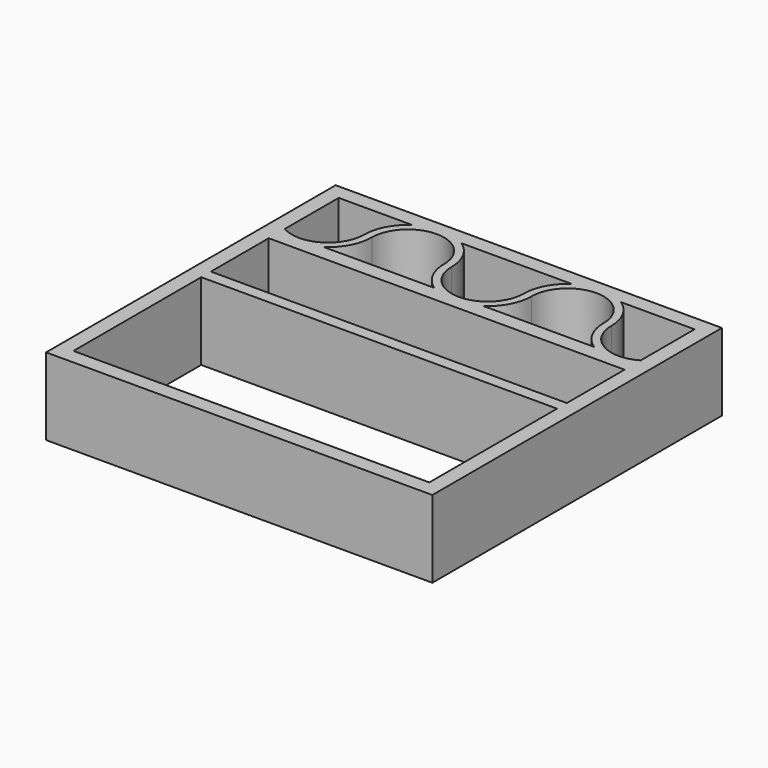
from build123d import *

# Parameters (mm, degrees)
F0_W     = 127
F0_H     = 119
F0_W_2   = 117
F0_H_2   = 23.75
F1_DEPTH = 25.4


# Not quite as in the source:
# - a feature of the source that left no trace in its solid (it failed there, or was rolled back) is left out


with BuildPart() as f1:
    # F0 (on Top) → F1 (new body)
    with BuildSketch(Plane.XY):
        Rectangle(F0_W, F0_H)
        Polygon((58.5, -54.5), (-58.5, -54.5), (-58.5, -30.75), (-58.5, -28.25), (-58.5, -25.75), (-58.5, -2), (58.5, -2), (58.5, -25.75), (58.5, -28.25), (58.5, -30.75), align=None, mode=Mode.SUBTRACT)
        with BuildLine():
            Line((-58.5, 32.3772868405), (-58.5, 54.5))
            Line((-58.5, 54.5), (-44.399074127, 54.5))
            Line((-44.399074127, 54.5), (-34.350925873, 54.5))
            ThreePointArc((-34.350925873, 54.5), (-38.9600636195, 49.3402742154), (-40.625, 42.625))
            ThreePointArc((-40.625, 42.625), (-46.5938326725, 32.3229219329), (-58.5, 32.3772868405))
        make_face(mode=Mode.SUBTRACT)
        with BuildLine():
            Line((-18.149074127, 30.75), (-44.399074127, 30.75))
            ThreePointArc((-44.399074127, 30.75), (-39.7899363805, 35.9097257846), (-38.125, 42.625))
            ThreePointArc((-38.125, 42.625), (-26.25, 54.5), (-14.375, 42.625))
            ThreePointArc((-14.375, 42.625), (-12.7100636195, 35.9097257846), (-8.100925873, 30.75))
            Line((-8.100925873, 30.75), (-18.149074127, 30.75))
        make_face(mode=Mode.SUBTRACT)
        with Locations((0, 13.875)):
            Rectangle(F0_W_2, F0_H_2, mode=Mode.SUBTRACT)
        with BuildLine():
            ThreePointArc((11.875, 42.625), (0, 30.75), (-11.875, 42.625))
            ThreePointArc((-11.875, 42.625), (-13.5399363805, 49.3402742154), (-18.149074127, 54.5))
            Line((-18.149074127, 54.5), (18.149074127, 54.5))
            ThreePointArc((18.149074127, 54.5), (13.5399363805, 49.3402742154), (11.875, 42.625))
        make_face(mode=Mode.SUBTRACT)
        with BuildLine():
            ThreePointArc((14.375, 42.625), (26.25, 54.5), (38.125, 42.625))
            ThreePointArc((38.125, 42.625), (39.7899363805, 35.9097257846), (44.399074127, 30.75))
            Line((44.399074127, 30.75), (8.100925873, 30.75))
            ThreePointArc((8.100925873, 30.75), (12.7100636195, 35.9097257846), (14.375, 42.625))
        make_face(mode=Mode.SUBTRACT)
        with BuildLine():
            Line((34.350925873, 54.5), (58.5, 54.5))
            Line((58.5, 54.5), (58.5, 32.3772868405))
            ThreePointArc((58.5, 32.3772868405), (46.5938326725, 32.3229219329), (40.625, 42.625))
            ThreePointArc((40.625, 42.625), (38.9600636195, 49.3402742154), (34.350925873, 54.5))
        make_face(mode=Mode.SUBTRACT)
    extrude(amount=F1_DEPTH)


solid = f1.part
